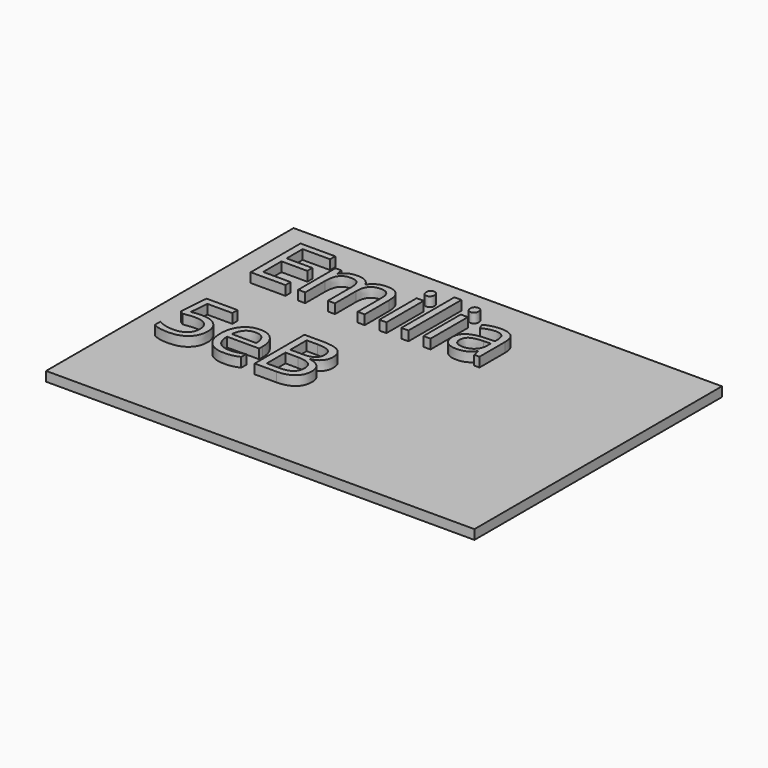
from build123d import *

# Parameters (mm, degrees)
F0_W         = 90
F0_H         = 65
F1_DEPTH     = 2
F2_TEXT_SIZE = 18.3287807482
F3_DEPTH     = 2


# Not quite as in the source:
# - Text() gives the source's letters only with a copy of the font that has no kerning and outlines rounded to 1/6400 em; it was checked with that copy


with BuildPart() as f1:
    # F0 (on Top) → F1 (new body)
    with BuildSketch(Plane.XY):
        with Locations((45, -32.5)):
            Rectangle(F0_W, F0_H)
    extrude(amount=F1_DEPTH)

    # F2 (on face) → F3 (join)
    with BuildSketch(Plane.XY.offset(2)):
        with Locations((4.9180341884, -19.6516402066)):
            Text('Emilia', F2_TEXT_SIZE, font='Open Sans', text_align=(TextAlign.LEFT, TextAlign.BOTTOM))
        with Locations((4.9180341884, -44.5787820241)):
            Text('5eB', F2_TEXT_SIZE, font='Open Sans', text_align=(TextAlign.LEFT, TextAlign.BOTTOM))
    extrude(amount=F3_DEPTH)


solid = f1.part
